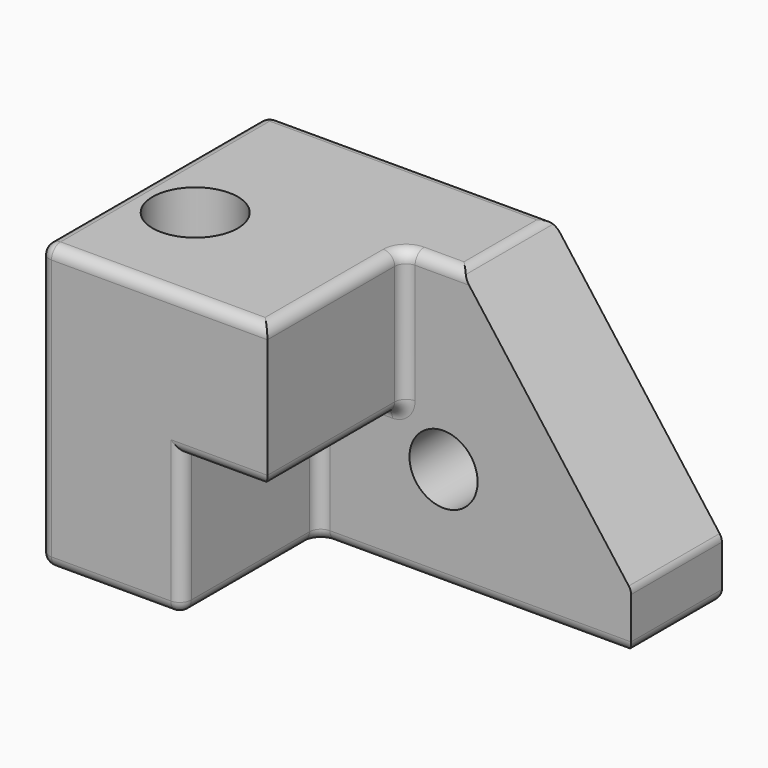
from build123d import *

# Parameters (mm, degrees)
F0_W     = 203.2
F0_H     = 127
F1_DEPTH = 127
F3_DEPTH = 76.2
F4_SIZE2 = 101.6
F4_SIZE  = 76.2
F5_R     = 5.08
F6_R     = 15.24
F7_DEPTH = 50.8
F8_R     = 19.05
F9_DEPTH = 127


with BuildPart() as f1:
    # F0 (on Front) → F1 (new body)
    with BuildSketch(Plane.XZ):
        with Locations((11.5803908557, 1.1079770926)):
            Rectangle(F0_W, F0_H)
    extrude(amount=F1_DEPTH)

    # F2 (on face) → F3 (cut)
    with BuildSketch(Plane.XZ.offset(127)):
        Polygon((-26.5196091443, 1.1079770926), (-26.5196091443, -62.3920229074), (113.1803908557, -62.3920229074), (113.1803908557, 64.6079770926), (11.5803908557, 64.6079770926), (11.5803908557, 1.1079770926), align=None)
    extrude(amount=-F3_DEPTH, mode=Mode.SUBTRACT)

    # F4
    f4_edges = [f1.edges().sort_by_distance(p)[0] for p in [
        (113.180391, -25.4, 64.607977),
    ]]
    f4_side = f1.faces().sort_by_distance((-10.191038, -52.614286, 64.607977))[0]
    chamfer(f4_edges, length=F4_SIZE, length2=F4_SIZE2, reference=f4_side)

    # F5
    f5_edges = [f1.edges().sort_by_distance(p)[0] for p in [
        (11.580391, -88.9, 64.607977),
        (11.580391, -88.9, 1.107977),
        (11.580391, -50.8, 32.857977),
        (-26.519609, -50.8, -30.642023),
        (-26.519609, -127, -30.642023),
        (-26.519609, -88.9, -62.392023),
        (-7.469609, -127, 1.107977),
        (-39.219609, -127, 64.607977),
        (-90.019609, -63.5, 64.607977),
        (-26.519609, 0, 64.607977),
        (-58.269609, -127, -62.392023),
        (-90.019609, -127, 1.107977),
        (43.330391, -50.8, -62.392023),
        (113.180391, -25.4, -62.392023),
        (36.980391, -25.4, 64.607977),
        (113.180391, -25.4, -36.992023),
        (11.580391, 0, -62.392023),
        (-90.019609, 0, 1.107977),
        (-90.019609, -63.5, -62.392023),
        (24.280391, -50.8, 64.607977),
        (-7.469609, -50.8, 1.107977),
    ]]
    fillet(f5_edges, radius=F5_R)

    # F6 (on face) → F7 (cut, through all)
    with BuildSketch(Plane.XZ.offset(50.8)):
        with Locations((29.3603908557, -16.6720229074)):
            Circle(F6_R)
    extrude(amount=-F7_DEPTH, mode=Mode.SUBTRACT)

    # F8 (on face) → F9 (cut)
    with BuildSketch(Plane.XY.offset(64.6079770926)):
        with Locations((-62.1130280197, -75.2307921648)):
            Circle(F8_R)
    extrude(amount=-F9_DEPTH, mode=Mode.SUBTRACT)


solid = f1.part
